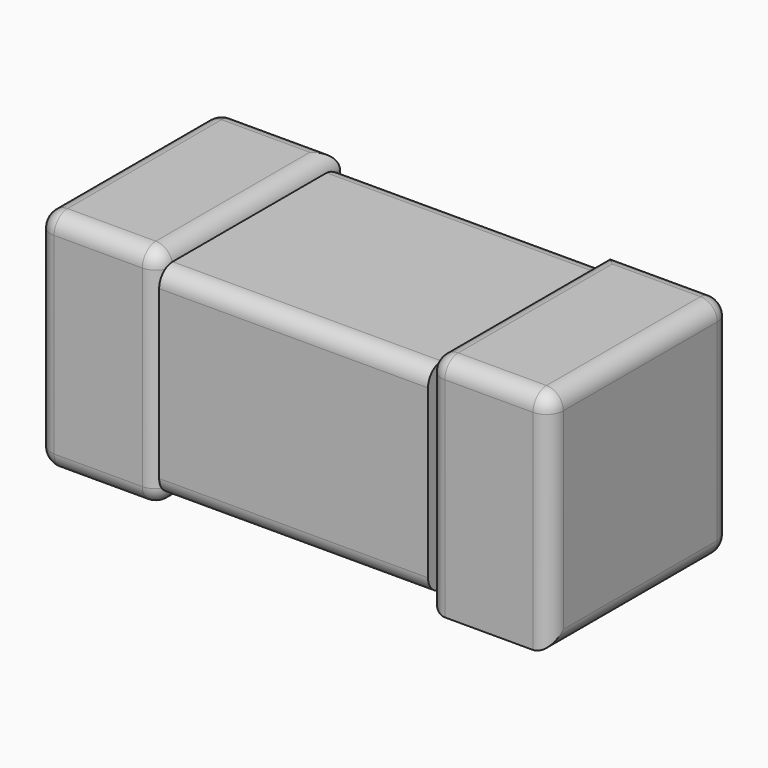
from build123d import *

# Parameters (mm, degrees)
F1_DEPTH = 1.345
F2_DEPTH = 1.345
F3_R     = 0.2
F3_2_R   = 0.2
F3_3_R   = 0.2


with BuildPart() as f1:
    # F0 (on Front) → F1 (new body, symmetric)
    with BuildSketch(Plane.XZ):
        Polygon((-1.6, 0), (-1.6, 0.15), (-1.6, 2.5396689307), (-1.6, 2.69), (-3.05, 2.69), (-3.05, 0), align=None)
    extrude(amount=F1_DEPTH, both=True)

    # F3#3
    f3_3_edges = [f1.edges().sort_by_distance(p)[0] for p in [
        (-3.05, 0, 0),
        (-3.05, -1.345, 1.345),
        (-3.05, 0, 2.69),
        (-3.05, 1.345, 1.345),
        (-2.325, 1.345, 0),
        (-2.325, -1.345, 0),
        (-1.6, -1.345, 1.345),
        (-1.6, 0, 0),
        (-2.325, -1.345, 2.69),
        (-1.6, 0, 2.69),
        (-2.325, 1.345, 2.69),
    ]]
    fillet(f3_3_edges, radius=F3_3_R)


with BuildPart() as f1b:
    # F0 (on Front) → F1, piece 2 (new body, symmetric)
    with BuildSketch(Plane.XZ):
        Polygon((1.6, 0.15), (1.6, 0), (3.05, 0), (3.05, 2.69), (1.6, 2.69), (1.6, 2.5396689307), align=None)
    extrude(amount=F1_DEPTH, both=True)

    # F3
    f3_edges = [f1b.edges().sort_by_distance(p)[0] for p in [
        (2.325, 1.345, 0),
        (3.05, 0, 0),
        (3.05, -1.345, 1.345),
        (3.05, 0, 2.69),
        (3.05, 1.345, 1.345),
        (2.325, 1.345, 2.69),
        (2.325, -1.345, 2.69),
        (1.6, -1.345, 1.345),
        (1.6, 0, 2.69),
        (1.6, 0, 0),
    ]]
    fillet(f3_edges, radius=F3_R)


with BuildPart() as f2:
    # F0 (on Front) → F2 (new body, symmetric)
    with BuildSketch(Plane.XZ):
        Polygon((0, 0.15), (1.6, 0.15), (1.6, 2.5396689307), (0, 2.5396689307), (-1.6, 2.5396689307), (-1.6, 0.15), align=None)
    extrude(amount=F2_DEPTH, both=True)

    # F3#2
    f3_2_edges = [f2.edges().sort_by_distance(p)[0] for p in [
        (0, -1.345, 2.539669),
        (0, -1.345, 0.15),
        (0, 1.345, 2.539669),
        (0, 1.345, 0.15),
        (-1.6, 1.345, 1.344834),
    ]]
    fillet(f3_2_edges, radius=F3_2_R)


solid = Compound([f1.part, f1b.part, f2.part])
